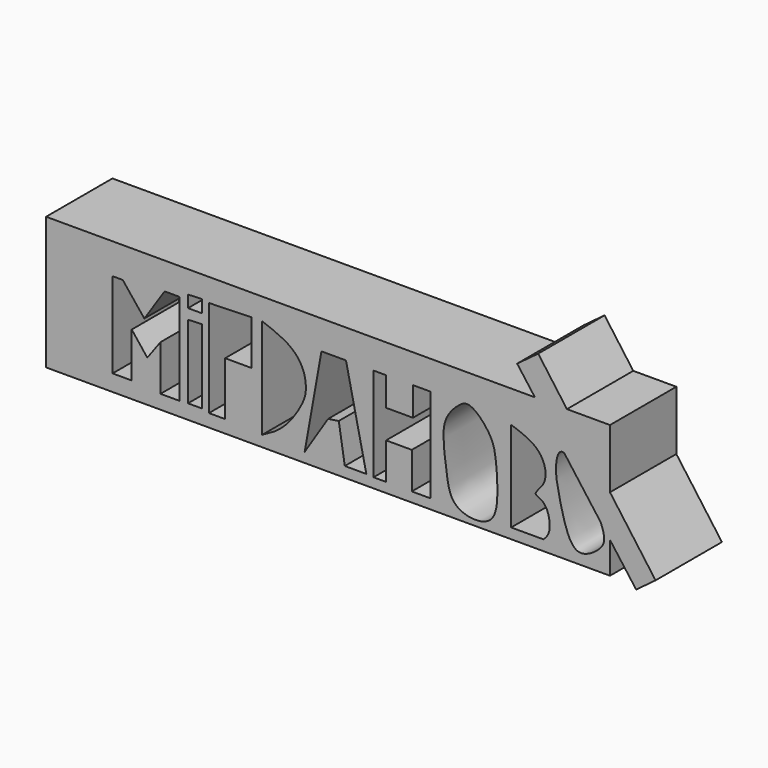
from build123d import *

# Parameters (mm, degrees)
F1_DEPTH = 25


with BuildPart() as f1:
    # F0 (on Front) → F1 (new body)
    with BuildSketch(Plane.XZ):
        with BuildLine():
            Line((62.3614487217, 20), (-85, 20))
            Line((-85, 20), (-85, -20))
            Line((-85, -20), (85, -20))
            Line((85, -20), (85, -10.4780528988))
            Line((85, -10.4780528988), (82.1477233246, -6.6380616235))
            add(Edge.make_bspline(
                [(70.7216560841, 8.2087628543), (69.1996240001, 8.2597046081), (68.3414146902, 2.5986308379), (69.4699440548, -2.6132865304), (70.92233283, -9.6987587114), (74.4703906649, -18.9967880488), (82.3791215508, -14.1877807655), (83.8699090457, -11.0948710225), (82.4150586587, -7.2636476642), (82.1477233246, -6.6380616235)],
                knots=[0, 0, 0, 0, 0.1155787502, 0.2389925832, 0.3780484198, 0.5193338278, 0.649131776, 0.7716422246, 0.793886795, 0.793886795, 0.793886795, 0.793886795], degree=3))
            add(Edge.make_bspline(
                [(71.1855970771, 8.1201382078), (71.0216461503, 8.1737580141), (70.8666294867, 8.2039106574), (70.7216560841, 8.2087628543)],
                knots=[0.9889911357, 0.9889911357, 0.9889911357, 0.9889911357, 1, 1, 1, 1], degree=3))
            Line((71.1855970771, 8.1201382078), (62.3614487217, 20))
        make_face()
        Polygon((-59.175260365, -15.064433217), (-64.9484544992, -15.064433217), (-64.9484544992, 10.734536685), (-61.8814490736, 10.734536685), (-55.3865991533, 2.615979407), (-49.2525808513, 11.8170101196), (-44.7422713041, 11.8170101196), (-44.7422713041, -15.7860834152), (-50.5154654384, -15.7860834152), (-50.5154654384, -2.0747422241), (-54.484538734, -7.4871135876), (-59.175260365, -1.533505274), align=None, mode=Mode.SUBTRACT)
        Polygon((-42.2164984047, -15.6056704), (-42.2164984047, 6.5850517713), (-38.0670130253, 6.7654643208), (-38.0670130253, -15.6056704), align=None, mode=Mode.SUBTRACT)
        Polygon((-35.9020642936, -16.1469075829), (-35.9020642936, 13.0798975006), (-23.0927839875, 13.4407216683), (-23.0927839875, 0), (-31.0309287161, 0), (-31.0309287161, -16.1469075829), align=None, mode=Mode.SUBTRACT)
        with BuildLine():
            Line((-19.8453627527, -16.6881456971), (-19.8453627527, 13.4407216683))
            add(Edge.make_bspline(
                [(-19.8453627527, -16.6881456971), (-17.7144681467, -15.59335519), (-13.1367992958, -13.2414845773), (-7.3969851182, -4.6052469009), (-6.3761514561, -0.138857195), (-7.3142777848, 5.5091079052), (-11.6998944818, 10.4400572546), (-16.984772428, 12.3869244765), (-19.8453627527, 13.4407216683)],
                knots=[0, 0, 0, 0, 0.174127985, 0.3740683612, 0.5092034405, 0.6544119692, 0.8129406606, 1, 1, 1, 1], degree=3))
        make_face(mode=Mode.SUBTRACT)
        Polygon((0, -6.0180414103), (-7.0360838436, -17.0489698648), (-1.9845368806, 11.275773868), (5.4123713635, 11.275773868), (11.5463910624, -16.868557781), (5.0515467301, -16.868557781), (3.247422399, -5.5025774054), align=None, mode=Mode.SUBTRACT)
        Polygon((13.7113435194, -17.0489698648), (13.7113435194, 11.275773868), (17.5000019372, 11.275773868), (17.5000019372, 2.615979407), (25.6185587496, 2.615979407), (25.6185587496, 11.275773868), (30.8505147696, 11.275773868), (30.8505147696, -17.0489698648), (25.2577345818, -17.0489698648), (25.2577345818, -6.0180414103), (17.5000019372, -6.0180414103), (17.5000019372, -17.0489698648), align=None, mode=Mode.SUBTRACT)
        with BuildLine():
            add(Edge.make_bspline(
                [(42.5773225725, 11.4561859518), (41.2511357888, 11.7931418797), (38.9387958075, 10.2842824948), (35.091033283, 5.9887509835), (34.5471614175, -0.1454559415), (35.716740771, -8.2593014734), (36.7995431786, -16.2955150436), (43.5529467814, -19.0002191266), (50.8997927145, -17.3629815935), (51.221081488, -7.2719863738), (50.6300974225, 0.0027132086), (49.5265289207, 5.6982324977), (44.5911531063, 10.9445143348), (42.5773225725, 11.4561859518)],
                knots=[0, 0, 0, 0, 0.0672415511, 0.1499170468, 0.2356057197, 0.3377976171, 0.4343645634, 0.5231992182, 0.6101239137, 0.7155971541, 0.8119871125, 0.8978928984, 1, 1, 1, 1], degree=3))
        make_face(mode=Mode.SUBTRACT)
        with BuildLine():
            Line((55.2061907947, -16.868557781), (55.2061907947, 10.373711586))
            add(Edge.make_bspline(
                [(64.9484544992, -16.868557781), (65.7243442417, -16.0570779127), (67.5818370767, -14.1143817299), (66.0112398073, -6.4637354468), (61.1283177948, -5.8607397386), (66.0833206675, -2.1457220786), (65.4791538436, 4.0353203529), (61.7276945752, 8.1338607507), (57.4755503841, 9.5942859898), (55.2061907947, 10.373711586)],
                knots=[0, 0, 0, 0, 0.121255707, 0.2902881616, 0.3988554907, 0.5298591304, 0.6843097284, 0.8315168271, 1, 1, 1, 1], degree=3))
            Line((64.9484544992, -16.868557781), (55.2061907947, -16.868557781))
        make_face(mode=Mode.SUBTRACT)
        Polygon((-42.2164984047, 9.6520623192), (-42.2164984047, 13.2603095844), (-38.0670130253, 13.4407216683), (-38.0670130253, 9.6520623192), align=None, mode=Mode.SUBTRACT)
        Polygon((57.0141535595, 27.1990094602), (62.3614487217, 20), (72.0245060165, 20), (63.3619472529, 31.9140368116), align=None)
        with BuildLine():
            Line((72.0245060165, 20), (62.3614487217, 20))
            Line((62.3614487217, 20), (71.1855970771, 8.1201382078))
            add(Edge.make_bspline(
                [(82.1477233246, -6.6380616235), (79.8029586036, -1.1511248386), (74.0912135488, 7.1698624433), (71.1855970771, 8.1201382078)],
                knots=[0.793886795, 0.793886795, 0.793886795, 0.793886795, 0.9889911357, 0.9889911357, 0.9889911357, 0.9889911357], degree=3))
            Line((82.1477233246, -6.6380616235), (85, -10.4780528988))
            Line((85, -10.4780528988), (85, 2.1541743973))
            Line((85, 2.1541743973), (72.0245060165, 20))
        make_face()
        Polygon((85, 20), (72.0245060165, 20), (85, 2.1541743973), align=None)
        with BuildLine():
            add(Edge.make_bspline(
                [(82.1477233246, -6.6380616235), (79.8029586036, -1.1511248386), (74.0912135488, 7.1698624433), (71.1855970771, 8.1201382078)],
                knots=[0.793886795, 0.793886795, 0.793886795, 0.793886795, 0.9889911357, 0.9889911357, 0.9889911357, 0.9889911357], degree=3))
            Line((71.1855970771, 8.1201382078), (82.1477233246, -6.6380616235))
        make_face()
        Polygon((98.7458772189, -16.751196598), (85, 2.1541743973), (85, -10.4780528988), (92.8902666326, -21.1006391613), align=None)
    extrude(amount=F1_DEPTH)


solid = f1.part
